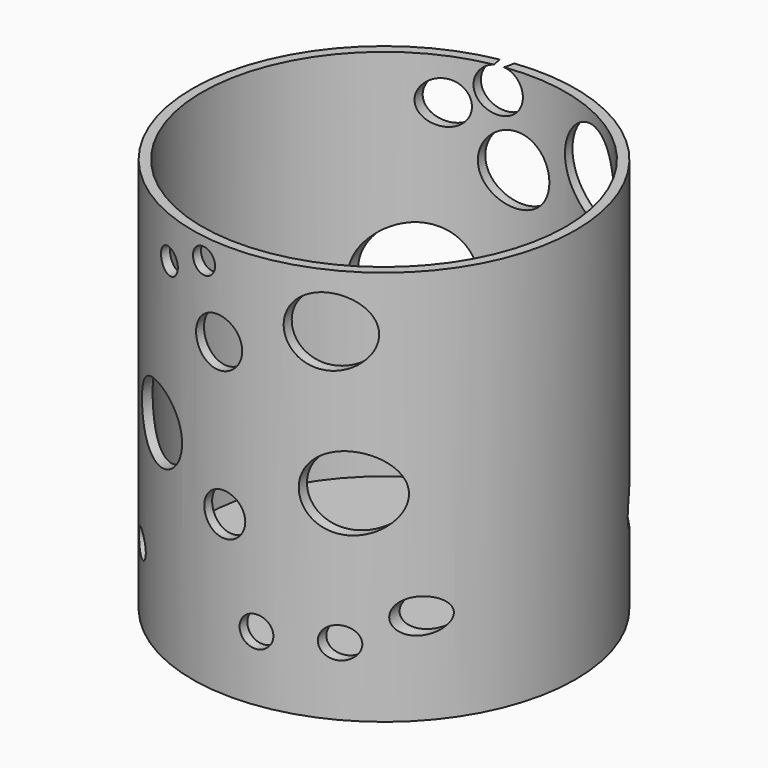
from build123d import *

# Parameters (mm, degrees)
F0_R     = 73.8583771587
F1_DEPTH = 152.4
F2_R     = 70.1167350622
F3_DEPTH = 144.018
F4_R     = 4.8364538457
F4_R_2   = 4.8423644085
F4_R_3   = 9.41220418
F4_R_4   = 14.2689032009
F4_R_5   = 13.9691522647
F4_R_6   = 13.228980881
F4_R_7   = 8.1345262345
F4_R_8   = 4.9068914895
F4_R_9   = 5.9065027345
F4_R_10  = 6.6489834961
F4_R_11  = 5.9930177398
F5_DEPTH = 117.348
F5_TAPER = -3
F6_DEPTH = 211.836


with BuildPart() as f1:
    # F0 (on Top) → F1 (new body)
    with BuildSketch(Plane.XY):
        Circle(F0_R)
    extrude(amount=F1_DEPTH)

    # F2 (on face) → F3 (cut)
    with BuildSketch(Plane.XY.offset(152.4)):
        Circle(F2_R)
    extrude(amount=-F3_DEPTH, mode=Mode.SUBTRACT)

    # F4 (on Front) → F5 (cut)
    with BuildSketch(Plane.XZ):
        with Locations((-11.0445292667, 144.1079974174)):
            Circle(F4_R)
        with Locations((-28.2631386071, 136.4552825689)):
            Circle(F4_R_2)
        with Locations((-5.0658448599, 118.7583804131)):
            Circle(F4_R_3)
        with Locations((37.5023819506, 77.1467387676)):
            Circle(F4_R_4)
        with Locations((-35.1984128356, 77.864177525)):
            Circle(F4_R_5)
        with Locations((31.7628495395, 131.4331889153)):
            Circle(F4_R_6)
        with Locations((-2.6743712369, 61.1238628626)):
            Circle(F4_R_7)
        with Locations((-49.7864000499, 28.1215272844)):
            Circle(F4_R_8)
        with Locations((9.2829959467, 25.0126104802)):
            Circle(F4_R_9)
        with Locations((54.0035516024, 35.5350933969)):
            Circle(F4_R_10)
        with Locations((34.8717644811, 26.2083504349)):
            Circle(F4_R_11)
    extrude(amount=-F5_DEPTH, taper=F5_TAPER, mode=Mode.SUBTRACT)

    # F4 (on Front) → F6 (cut)
    with BuildSketch(Plane.XZ):
        with Locations((-11.0445292667, 144.1079974174)):
            Circle(F4_R)
        with Locations((-28.2631386071, 136.4552825689)):
            Circle(F4_R_2)
        with Locations((-5.0658448599, 118.7583804131)):
            Circle(F4_R_3)
        with Locations((37.5023819506, 77.1467387676)):
            Circle(F4_R_4)
        with Locations((-35.1984128356, 77.864177525)):
            Circle(F4_R_5)
        with Locations((31.7628495395, 131.4331889153)):
            Circle(F4_R_6)
        with Locations((-2.6743712369, 61.1238628626)):
            Circle(F4_R_7)
        with Locations((-49.7864000499, 28.1215272844)):
            Circle(F4_R_8)
        with Locations((9.2829959467, 25.0126104802)):
            Circle(F4_R_9)
        with Locations((54.0035516024, 35.5350933969)):
            Circle(F4_R_10)
        with Locations((34.8717644811, 26.2083504349)):
            Circle(F4_R_11)
    extrude(amount=F6_DEPTH, mode=Mode.SUBTRACT)


solid = f1.part
